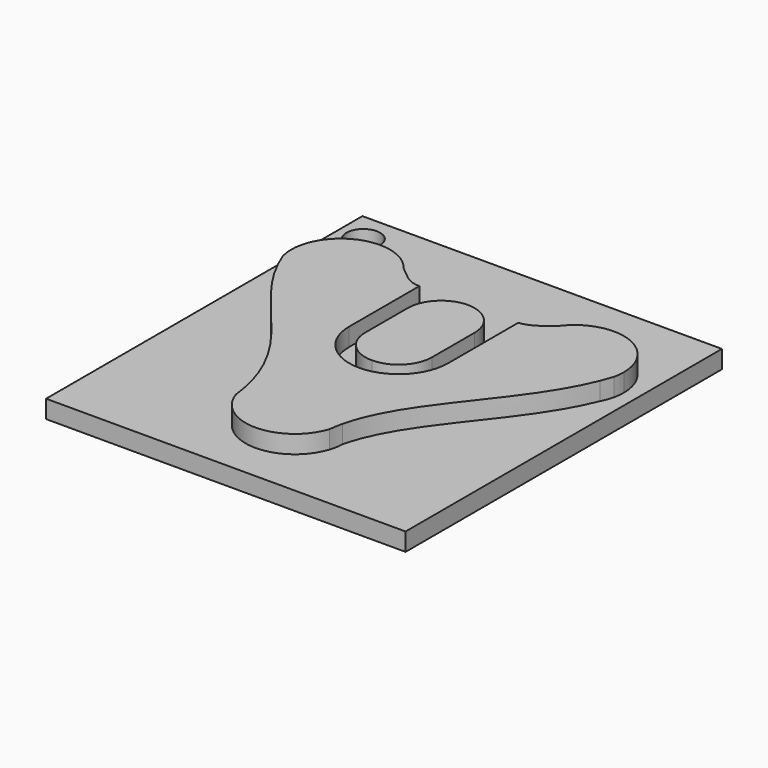
from build123d import *

# Parameters (mm, degrees)
F0_W     = 50
F0_H     = 55
F0_R     = 2.3365962568
F1_DEPTH = 2.5
F2_DEPTH = 2.5


with BuildPart() as f1:
    # F0 (on Top) → F1 (new body)
    with BuildSketch(Plane.XY):
        with Locations((0, 12.341101347)):
            Rectangle(F0_W, F0_H)
        with BuildLine():
            ThreePointArc((10.8052556607, 29.2671544041), (18.4488604009, 31.6259838811), (23.1186818497, 25.1312523575))
            ThreePointArc((23.1186818497, 25.1312523575), (23.0790338974, 24.3952437271), (22.9605489193, 23.6677535387))
            ThreePointArc((22.9605489193, 23.6677535387), (22.7111144002, 22.8034574753), (22.3505935824, 21.9792912273))
            add(Edge.make_bspline(
                [(22.3505935824, 21.9792912273), (18.484972418, 12.3846041121), (8.9944482287, 5.6182022343), (6.8467520485, -3.4005596444)],
                knots=[1.7047136512, 1.7047136512, 1.7047136512, 1.7047136512, 31.2766934929, 31.2766934929, 31.2766934929, 31.2766934929], degree=3))
            ThreePointArc((6.8467520485, -3.4005596444), (6.7459359262, -4.3477283467), (6.5147303328, -5.271761038))
            ThreePointArc((6.5147303328, -5.271761038), (0, -10.0020528135), (-6.5147303328, -5.271761038))
            ThreePointArc((-6.5147303328, -5.271761038), (-6.7668462793, -4.2232244294), (-6.851307477, -3.1481161668))
            add(Edge.make_bspline(
                [(-22.1192262656, 21.568073359), (-17.9179549259, 12.7340303131), (-9.0631935188, 7.6895660109), (-6.851307477, -3.1481161668)],
                knots=[1.9402705078, 1.9402705078, 1.9402705078, 1.9402705078, 31.1584988533, 31.1584988533, 31.1584988533, 31.1584988533], degree=3))
            ThreePointArc((-22.1192262656, 21.568073359), (-22.57078803, 22.4465939133), (-22.8913266517, 23.3809179381))
            ThreePointArc((-22.8913266517, 23.3809179381), (-19.2672755049, 31.2908798808), (-10.8052556607, 29.2671544041))
            add(Edge.make_bspline(
                [(-10.8052556607, 29.2671544041), (-9.3004167648, 28.0267296842), (-8.4820119868, 27.09910709), (-6.8878750083, 27.09910709)],
                knots=[0, 0, 0, 0, 4.4773094971, 4.4773094971, 4.4773094971, 4.4773094971], degree=3))
            Line((-6.8878750083, 27.09910709), (-6.8878750083, 14.8940041956))
            ThreePointArc((-6.8878750083, 14.8940041956), (0, 8.0061291873), (6.8878750083, 14.8940041956))
            Line((6.8878750083, 14.8940041956), (6.8878750083, 27.09910709))
            add(Edge.make_bspline(
                [(10.8052556607, 29.2671544041), (9.4734053303, 28.0257134136), (8.0485488803, 27.09910709), (6.8878750083, 27.09910709)],
                knots=[0, 0, 0, 0, 4.4773094971, 4.4773094971, 4.4773094971, 4.4773094971], degree=3))
        make_face(mode=Mode.SUBTRACT)
        with Locations((-21.5719379485, 35.7079468668)):
            Circle(F0_R, mode=Mode.SUBTRACT)
        with BuildLine():
            ThreePointArc((-4.6471344177, 22.2825248368), (0, 26.9296592545), (4.6471344177, 22.2825248368))
            Line((4.6471344177, 22.2825248368), (4.6471344177, 14.8940041956))
            ThreePointArc((4.6471344177, 14.8940041956), (3.2860202598, 11.6079839357), (0, 10.2468697779))
            ThreePointArc((0, 10.2468697779), (-3.2860202598, 11.6079839357), (-4.6471344177, 14.8940041956))
            Line((-4.6471344177, 14.8940041956), (-4.6471344177, 22.2825248368))
        make_face(mode=Mode.SUBTRACT)
        with BuildLine():
            ThreePointArc((22.3505935824, 21.9792912273), (12.6102330192, 19.3376574577), (10.8052556607, 29.2671544041))
            add(Edge.make_bspline(
                [(10.8052556607, 29.2671544041), (9.4734053303, 28.0257134136), (8.0485488803, 27.09910709), (6.8878750083, 27.09910709)],
                knots=[0, 0, 0, 0, 4.4773094971, 4.4773094971, 4.4773094971, 4.4773094971], degree=3))
            Line((6.8878750083, 27.09910709), (6.8878750083, 14.8940041956))
            ThreePointArc((6.8878750083, 14.8940041956), (0, 8.0061291873), (-6.8878750083, 14.8940041956))
            Line((-6.8878750083, 14.8940041956), (-6.8878750083, 27.09910709))
            add(Edge.make_bspline(
                [(-10.8052556607, 29.2671544041), (-9.3004167648, 28.0267296842), (-8.4820119868, 27.09910709), (-6.8878750083, 27.09910709)],
                knots=[0, 0, 0, 0, 4.4773094971, 4.4773094971, 4.4773094971, 4.4773094971], degree=3))
            ThreePointArc((-10.8052556607, 29.2671544041), (-9.7726423449, 27.31273889), (-9.4160658872, 25.1312523575))
            ThreePointArc((-9.4160658872, 25.1312523575), (-14.4170255201, 18.5345386269), (-22.1192262656, 21.568073359))
            add(Edge.make_bspline(
                [(-22.1192262656, 21.568073359), (-17.9179549259, 12.7340303131), (-9.0631935188, 7.6895660109), (-6.851307477, -3.1481161668)],
                knots=[1.9402705078, 1.9402705078, 1.9402705078, 1.9402705078, 31.1584988533, 31.1584988533, 31.1584988533, 31.1584988533], degree=3))
            ThreePointArc((-6.851307477, -3.1481161668), (0.0013143327, 3.700563023), (6.8513079813, -3.1507448322))
            ThreePointArc((6.8513079813, -3.1507448322), (6.8501689034, -3.2756730085), (6.8467520485, -3.4005596444))
            add(Edge.make_bspline(
                [(22.3505935824, 21.9792912273), (18.484972418, 12.3846041121), (8.9944482287, 5.6182022343), (6.8467520485, -3.4005596444)],
                knots=[1.7047136512, 1.7047136512, 1.7047136512, 1.7047136512, 31.2766934929, 31.2766934929, 31.2766934929, 31.2766934929], degree=3))
        make_face()
        with BuildLine():
            ThreePointArc((22.9605489193, 23.6677535387), (23.0790338974, 24.3952437271), (23.1186818497, 25.1312523575))
            ThreePointArc((23.1186818497, 25.1312523575), (18.4488604009, 31.6259838811), (10.8052556607, 29.2671544041))
            ThreePointArc((10.8052556607, 29.2671544041), (12.6102330192, 19.3376574577), (22.3505935824, 21.9792912273))
            add(Edge.make_bspline(
                [(22.9605489193, 23.6677535387), (22.7775786287, 23.0948852778), (22.5734321344, 22.5323889297), (22.3505935824, 21.9792912273)],
                knots=[0, 0, 0, 0, 1.7047136512, 1.7047136512, 1.7047136512, 1.7047136512], degree=3))
        make_face()
        with BuildLine():
            add(Edge.make_bspline(
                [(-22.8913266517, 23.3809179381), (-22.6566860437, 22.7580544126), (-22.3982165856, 22.1547082838), (-22.1192262656, 21.568073359)],
                knots=[0, 0, 0, 0, 1.9402705078, 1.9402705078, 1.9402705078, 1.9402705078], degree=3))
            ThreePointArc((-22.1192262656, 21.568073359), (-14.4170255201, 18.5345386269), (-9.4160658872, 25.1312523575))
            ThreePointArc((-9.4160658872, 25.1312523575), (-9.7726423449, 27.31273889), (-10.8052556607, 29.2671544041))
            ThreePointArc((-10.8052556607, 29.2671544041), (-19.2672755049, 31.2908798808), (-22.8913266517, 23.3809179381))
        make_face()
        with BuildLine():
            add(Edge.make_bspline(
                [(6.8467520485, -3.4005596444), (6.7008211488, -4.0133632838), (6.5887912239, -4.6365658048), (6.5147303328, -5.271761038)],
                knots=[31.2766934929, 31.2766934929, 31.2766934929, 31.2766934929, 33.2860399103, 33.2860399103, 33.2860399103, 33.2860399103], degree=3))
            ThreePointArc((6.8467520485, -3.4005596444), (6.8501689034, -3.2756730085), (6.8513079813, -3.1507448322))
            ThreePointArc((6.8513079813, -3.1507448322), (0.0013143327, 3.700563023), (-6.851307477, -3.1481161668))
            add(Edge.make_bspline(
                [(-6.851307477, -3.1481161668), (-6.7117079268, -3.8321186553), (-6.5985689132, -4.5391972434), (-6.5147303328, -5.271761038)],
                knots=[31.1584988533, 31.1584988533, 31.1584988533, 31.1584988533, 33.0025592871, 33.0025592871, 33.0025592871, 33.0025592871], degree=3))
            ThreePointArc((-6.5147303328, -5.271761038), (0, -10.0020528135), (6.5147303328, -5.271761038))
        make_face()
        with BuildLine():
            ThreePointArc((2.819272775, 18.5882645162), (4.1651769375, 20.2216610918), (4.6471344177, 22.2825248368))
            ThreePointArc((4.6471344177, 22.2825248368), (0, 26.9296592545), (-4.6471344177, 22.2825248368))
            ThreePointArc((-4.6471344177, 22.2825248368), (-4.1651769375, 20.2216610918), (-2.819272775, 18.5882645162))
            ThreePointArc((-2.819272775, 18.5882645162), (0, 19.5411386133), (2.819272775, 18.5882645162))
        make_face()
        with BuildLine():
            ThreePointArc((4.6471344177, 14.8940041956), (4.1651769375, 16.9548679405), (2.819272775, 18.5882645162))
            ThreePointArc((2.819272775, 18.5882645162), (1.4879741282, 17.8800492502), (0, 17.6353904191))
            Line((0, 17.6353904191), (0, 10.2468697779))
            ThreePointArc((0, 10.2468697779), (3.2860202598, 11.6079839357), (4.6471344177, 14.8940041956))
        make_face()
        with BuildLine():
            ThreePointArc((0, 17.6353904191), (-1.4879741282, 17.8800492502), (-2.819272775, 18.5882645162))
            ThreePointArc((-2.819272775, 18.5882645162), (-4.1651769375, 16.9548679405), (-4.6471344177, 14.8940041956))
            ThreePointArc((-4.6471344177, 14.8940041956), (-3.2860202598, 11.6079839357), (0, 10.2468697779))
            Line((0, 10.2468697779), (0, 17.6353904191))
        make_face()
        with BuildLine():
            ThreePointArc((0, 17.6353904191), (1.4879741282, 17.8800492502), (2.819272775, 18.5882645162))
            ThreePointArc((2.819272775, 18.5882645162), (0, 19.5411386133), (-2.819272775, 18.5882645162))
            ThreePointArc((-2.819272775, 18.5882645162), (-1.4879741282, 17.8800492502), (0, 17.6353904191))
        make_face()
        with BuildLine():
            Line((4.6471344177, 14.8940041956), (4.6471344177, 22.2825248368))
            ThreePointArc((4.6471344177, 22.2825248368), (4.1651769375, 20.2216610918), (2.819272775, 18.5882645162))
            ThreePointArc((2.819272775, 18.5882645162), (4.1651769375, 16.9548679405), (4.6471344177, 14.8940041956))
        make_face()
        with BuildLine():
            ThreePointArc((-2.819272775, 18.5882645162), (-4.1651769375, 20.2216610918), (-4.6471344177, 22.2825248368))
            Line((-4.6471344177, 22.2825248368), (-4.6471344177, 14.8940041956))
            ThreePointArc((-4.6471344177, 14.8940041956), (-4.1651769375, 16.9548679405), (-2.819272775, 18.5882645162))
        make_face()
    extrude(amount=-F1_DEPTH)

    # F0 (on Top) → F2 (join)
    with BuildSketch(Plane.XY):
        with BuildLine():
            ThreePointArc((2.819272775, 18.5882645162), (4.1651769375, 20.2216610918), (4.6471344177, 22.2825248368))
            ThreePointArc((4.6471344177, 22.2825248368), (0, 26.9296592545), (-4.6471344177, 22.2825248368))
            ThreePointArc((-4.6471344177, 22.2825248368), (-4.1651769375, 20.2216610918), (-2.819272775, 18.5882645162))
            ThreePointArc((-2.819272775, 18.5882645162), (0, 19.5411386133), (2.819272775, 18.5882645162))
        make_face()
        with BuildLine():
            Line((4.6471344177, 14.8940041956), (4.6471344177, 22.2825248368))
            ThreePointArc((4.6471344177, 22.2825248368), (4.1651769375, 20.2216610918), (2.819272775, 18.5882645162))
            ThreePointArc((2.819272775, 18.5882645162), (4.1651769375, 16.9548679405), (4.6471344177, 14.8940041956))
        make_face()
        with BuildLine():
            ThreePointArc((-2.819272775, 18.5882645162), (-4.1651769375, 20.2216610918), (-4.6471344177, 22.2825248368))
            Line((-4.6471344177, 22.2825248368), (-4.6471344177, 14.8940041956))
            ThreePointArc((-4.6471344177, 14.8940041956), (-4.1651769375, 16.9548679405), (-2.819272775, 18.5882645162))
        make_face()
        with BuildLine():
            ThreePointArc((4.6471344177, 14.8940041956), (4.1651769375, 16.9548679405), (2.819272775, 18.5882645162))
            ThreePointArc((2.819272775, 18.5882645162), (1.4879741282, 17.8800492502), (0, 17.6353904191))
            Line((0, 17.6353904191), (0, 10.2468697779))
            ThreePointArc((0, 10.2468697779), (3.2860202598, 11.6079839357), (4.6471344177, 14.8940041956))
        make_face()
        with BuildLine():
            ThreePointArc((0, 17.6353904191), (1.4879741282, 17.8800492502), (2.819272775, 18.5882645162))
            ThreePointArc((2.819272775, 18.5882645162), (0, 19.5411386133), (-2.819272775, 18.5882645162))
            ThreePointArc((-2.819272775, 18.5882645162), (-1.4879741282, 17.8800492502), (0, 17.6353904191))
        make_face()
        with BuildLine():
            ThreePointArc((0, 17.6353904191), (-1.4879741282, 17.8800492502), (-2.819272775, 18.5882645162))
            ThreePointArc((-2.819272775, 18.5882645162), (-4.1651769375, 16.9548679405), (-4.6471344177, 14.8940041956))
            ThreePointArc((-4.6471344177, 14.8940041956), (-3.2860202598, 11.6079839357), (0, 10.2468697779))
            Line((0, 10.2468697779), (0, 17.6353904191))
        make_face()
        with BuildLine():
            ThreePointArc((22.9605489193, 23.6677535387), (23.0790338974, 24.3952437271), (23.1186818497, 25.1312523575))
            ThreePointArc((23.1186818497, 25.1312523575), (18.4488604009, 31.6259838811), (10.8052556607, 29.2671544041))
            ThreePointArc((10.8052556607, 29.2671544041), (12.6102330192, 19.3376574577), (22.3505935824, 21.9792912273))
            add(Edge.make_bspline(
                [(22.9605489193, 23.6677535387), (22.7775786287, 23.0948852778), (22.5734321344, 22.5323889297), (22.3505935824, 21.9792912273)],
                knots=[0, 0, 0, 0, 1.7047136512, 1.7047136512, 1.7047136512, 1.7047136512], degree=3))
        make_face()
        with BuildLine():
            ThreePointArc((22.3505935824, 21.9792912273), (12.6102330192, 19.3376574577), (10.8052556607, 29.2671544041))
            add(Edge.make_bspline(
                [(10.8052556607, 29.2671544041), (9.4734053303, 28.0257134136), (8.0485488803, 27.09910709), (6.8878750083, 27.09910709)],
                knots=[0, 0, 0, 0, 4.4773094971, 4.4773094971, 4.4773094971, 4.4773094971], degree=3))
            Line((6.8878750083, 27.09910709), (6.8878750083, 14.8940041956))
            ThreePointArc((6.8878750083, 14.8940041956), (0, 8.0061291873), (-6.8878750083, 14.8940041956))
            Line((-6.8878750083, 14.8940041956), (-6.8878750083, 27.09910709))
            add(Edge.make_bspline(
                [(-10.8052556607, 29.2671544041), (-9.3004167648, 28.0267296842), (-8.4820119868, 27.09910709), (-6.8878750083, 27.09910709)],
                knots=[0, 0, 0, 0, 4.4773094971, 4.4773094971, 4.4773094971, 4.4773094971], degree=3))
            ThreePointArc((-10.8052556607, 29.2671544041), (-9.7726423449, 27.31273889), (-9.4160658872, 25.1312523575))
            ThreePointArc((-9.4160658872, 25.1312523575), (-14.4170255201, 18.5345386269), (-22.1192262656, 21.568073359))
            add(Edge.make_bspline(
                [(-22.1192262656, 21.568073359), (-17.9179549259, 12.7340303131), (-9.0631935188, 7.6895660109), (-6.851307477, -3.1481161668)],
                knots=[1.9402705078, 1.9402705078, 1.9402705078, 1.9402705078, 31.1584988533, 31.1584988533, 31.1584988533, 31.1584988533], degree=3))
            ThreePointArc((-6.851307477, -3.1481161668), (0.0013143327, 3.700563023), (6.8513079813, -3.1507448322))
            ThreePointArc((6.8513079813, -3.1507448322), (6.8501689034, -3.2756730085), (6.8467520485, -3.4005596444))
            add(Edge.make_bspline(
                [(22.3505935824, 21.9792912273), (18.484972418, 12.3846041121), (8.9944482287, 5.6182022343), (6.8467520485, -3.4005596444)],
                knots=[1.7047136512, 1.7047136512, 1.7047136512, 1.7047136512, 31.2766934929, 31.2766934929, 31.2766934929, 31.2766934929], degree=3))
        make_face()
        with BuildLine():
            add(Edge.make_bspline(
                [(6.8467520485, -3.4005596444), (6.7008211488, -4.0133632838), (6.5887912239, -4.6365658048), (6.5147303328, -5.271761038)],
                knots=[31.2766934929, 31.2766934929, 31.2766934929, 31.2766934929, 33.2860399103, 33.2860399103, 33.2860399103, 33.2860399103], degree=3))
            ThreePointArc((6.8467520485, -3.4005596444), (6.8501689034, -3.2756730085), (6.8513079813, -3.1507448322))
            ThreePointArc((6.8513079813, -3.1507448322), (0.0013143327, 3.700563023), (-6.851307477, -3.1481161668))
            add(Edge.make_bspline(
                [(-6.851307477, -3.1481161668), (-6.7117079268, -3.8321186553), (-6.5985689132, -4.5391972434), (-6.5147303328, -5.271761038)],
                knots=[31.1584988533, 31.1584988533, 31.1584988533, 31.1584988533, 33.0025592871, 33.0025592871, 33.0025592871, 33.0025592871], degree=3))
            ThreePointArc((-6.5147303328, -5.271761038), (0, -10.0020528135), (6.5147303328, -5.271761038))
        make_face()
        with BuildLine():
            add(Edge.make_bspline(
                [(-22.8913266517, 23.3809179381), (-22.6566860437, 22.7580544126), (-22.3982165856, 22.1547082838), (-22.1192262656, 21.568073359)],
                knots=[0, 0, 0, 0, 1.9402705078, 1.9402705078, 1.9402705078, 1.9402705078], degree=3))
            ThreePointArc((-22.1192262656, 21.568073359), (-14.4170255201, 18.5345386269), (-9.4160658872, 25.1312523575))
            ThreePointArc((-9.4160658872, 25.1312523575), (-9.7726423449, 27.31273889), (-10.8052556607, 29.2671544041))
            ThreePointArc((-10.8052556607, 29.2671544041), (-19.2672755049, 31.2908798808), (-22.8913266517, 23.3809179381))
        make_face()
    extrude(amount=F2_DEPTH)


solid = f1.part
